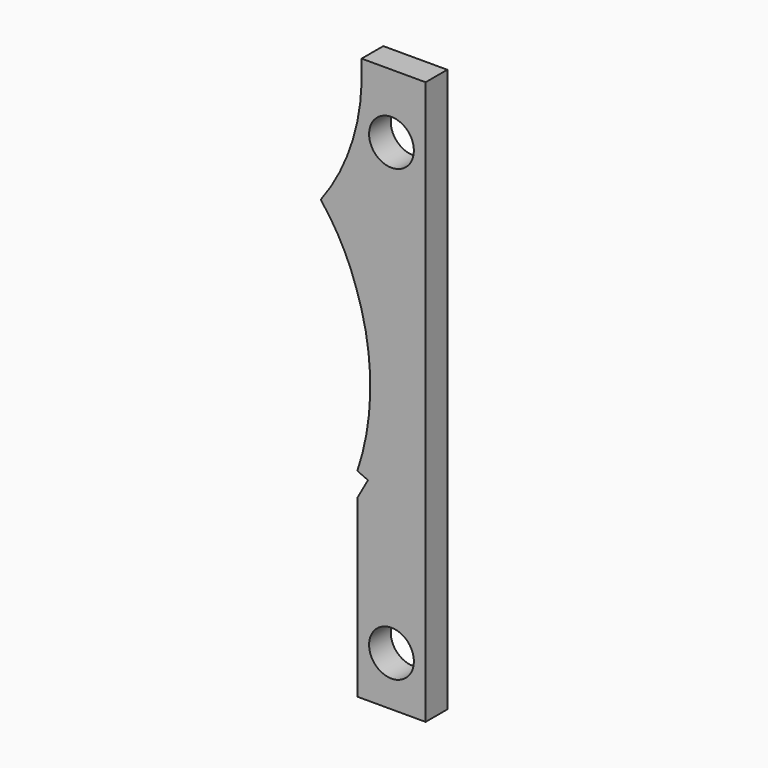
from build123d import *

# Parameters (mm, degrees)
F0_R     = 5.2500022
F1_DEPTH = 6.35


# Not quite as in the source:
# - ends of sketch curves that miss each other by under 0.0002 mm in the source are joined


with BuildPart() as f1:
    # F0 (on Front) → F1 (new body)
    with BuildSketch(Plane.XZ):
        with BuildLine():
            Line((-2.7092148, 65.999995), (-2.7092148, 60.9999796))
            ThreePointArc((-2.7092148, 60.9999796), (-5.4016290161, 46.6516213468), (-12.2907672961, 33.7805612895))
            ThreePointArc((-12.2907672961, 33.7805612895), (-7.426360466, 26.392264731), (-3.9728687393, 18.248400136))
            ThreePointArc((-3.9728687393, 18.248400136), (-0.6755780926, -0.5535614771), (-3.7092166309, -19.3998583041))
            Line((-3.7092166309, -19.3998583041), (-1.2092178, -20.5000098))
            Line((-1.2092178, -20.5000098), (-3.7092128, -24.9706384))
            Line((-3.7092128, -24.9706384), (-3.7092128, -65.999995))
            Line((-3.7092128, -65.999995), (12.2907806, -65.999995))
            Line((12.2907806, -65.999995), (12.2907806, 65.999995))
            Line((12.2907806, 65.999995), (-2.7092148, 65.999995))
        make_face()
        with Locations((4.2907712, -54.4085272)):
            Circle(F0_R, mode=Mode.SUBTRACT)
        with Locations((4.2907712, 50.9999996)):
            Circle(F0_R, mode=Mode.SUBTRACT)
    extrude(amount=F1_DEPTH)


solid = f1.part
